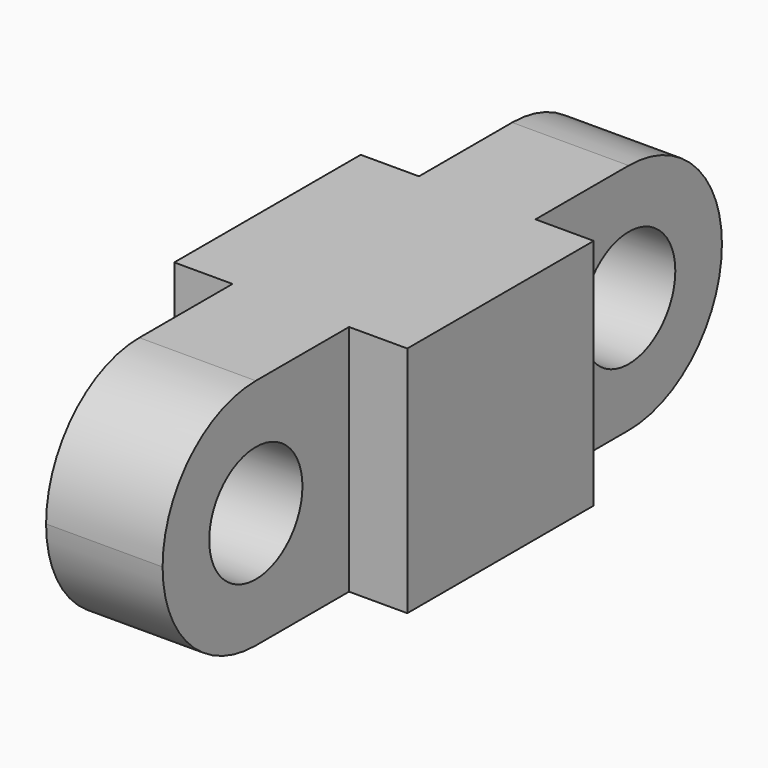
from build123d import *

# Parameters (mm, degrees)
F1_DEPTH = 40
F3_DEPTH = 20
F4_R     = 19.99999
F5_R     = 10
F6_DEPTH = 25


# Not quite as in the source:
# - a fillet or chamfer is up to 0.001 mm smaller than in the source, because OpenCascade refuses the exact size


with BuildPart() as f1:
    # F0 (on Top) → F1 (new body)
    with BuildSketch(Plane.XY):
        Polygon((10, 40), (10, 0), (30, 0), (30, 40), (40, 40), (40, 80), (30, 80), (30, 120), (10, 120), (10, 80), (0, 80), (0, 40), align=None)
    extrude(amount=F1_DEPTH)

    # F2 (on face) → F3 (cut)
    with BuildSketch(Plane.YZ.offset(30)):
        with BuildLine():
            ThreePointArc((20, 0), (5.8578643763, 5.8578643763), (0, 20))
            Line((0, 20), (0, 0))
            Line((0, 0), (20, 0))
        make_face()
        with BuildLine():
            ThreePointArc((0, 20), (5.8578643763, 34.1421356237), (20, 40))
            Line((20, 40), (0, 40))
            Line((0, 40), (0, 20))
        make_face()
    extrude(amount=-F3_DEPTH, mode=Mode.SUBTRACT)

    # F4 (radius 20 in the source; OpenCascade refuses exactly that, so slightly less here)
    f4_edges = [f1.edges().sort_by_distance(p)[0] for p in [
        (20, 120, 0),
        (20, 120, 40),
    ]]
    fillet(f4_edges, radius=F4_R)

    # F5 (on face) → F6 (cut)
    with BuildSketch(Plane.YZ.offset(30)):
        with Locations((100, 20)):
            Circle(F5_R)
        with Locations((20, 20)):
            Circle(F5_R)
    extrude(amount=-F6_DEPTH, mode=Mode.SUBTRACT)


solid = f1.part
